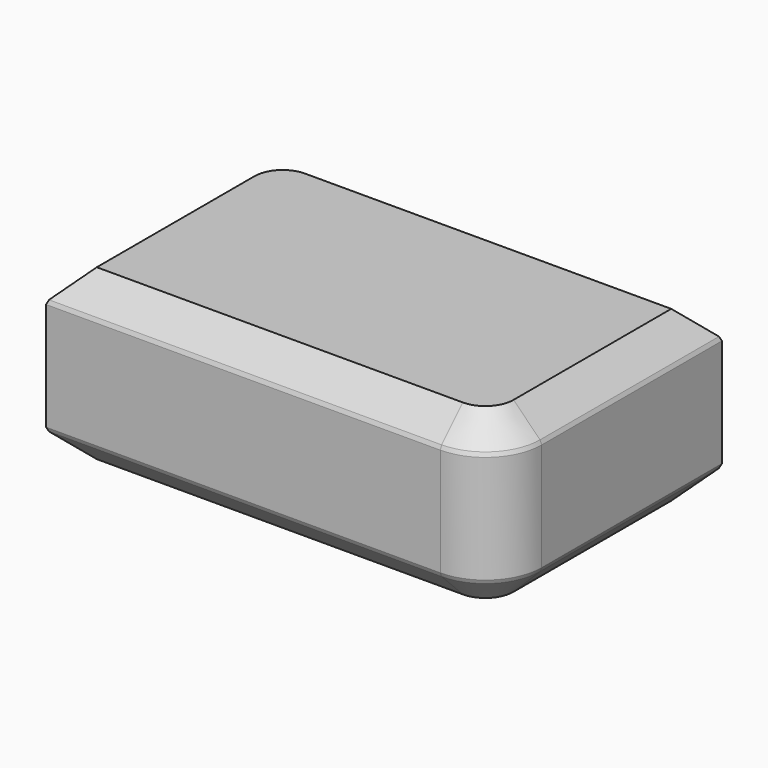
from build123d import *

# Parameters (mm, degrees)
F1_DEPTH     = 76.2
F2_SIZE      = 12.7
F3_T1_DEPTH  = 180.6665699849
F3_T3_DEPTH  = 104.4665699849
F3_T5_DEPTH  = 104.4665699849
F3_T7_DEPTH  = 180.6665699849
F3_T10_ANGLE = 90
F3_T12_ANGLE = 90
F3_T14_ANGLE = 90
F3_T16_ANGLE = 90


# Not quite as in the source:
# - a fillet or chamfer that OpenCascade refuses, or shapes differently, is made with other operations: its cross-section is extruded or revolved along the edge and cut away or added


with BuildPart() as f1:
    # F0 (on Top) → F1 (new body)
    with BuildSketch(Plane.XY):
        with BuildLine():
            Line((137.0133969558, 56.4750247419), (-40.7866030442, 56.4750247419))
            ThreePointArc((-40.7866030442, 56.4750247419), (-58.7471152864, 49.035536984), (-66.1866030442, 31.0750247419))
            Line((-66.1866030442, 31.0750247419), (-66.1866030442, -70.5249752581))
            Line((-66.1866030442, -70.5249752581), (111.6133969558, -70.5249752581))
            ThreePointArc((111.6133969558, -70.5249752581), (129.5739091979, -63.0854875003), (137.0133969558, -45.1249752581))
            Line((137.0133969558, -45.1249752581), (137.0133969558, 56.4750247419))
        make_face()
    extrude(amount=F1_DEPTH)

    # F2
    f2_edges = [f1.edges().sort_by_distance(p)[0] for p in [
        (48.113397, 56.475025, 76.2),
        (-58.747115, 49.035537, 76.2),
        (-66.186603, -19.724975, 76.2),
        (22.713397, -70.524975, 76.2),
        (129.573909, -63.085488, 76.2),
        (137.013397, 5.675025, 76.2),
        (48.113397, 56.475025, 0),
        (-58.747115, 49.035537, 0),
        (-66.186603, -19.724975, 0),
        (22.713397, -70.524975, 0),
        (129.573909, -63.085488, 0),
        (137.013397, 5.675025, 0),
    ]]
    chamfer(f2_edges, length=F2_SIZE)

    # F3: chamfer of 2.54 on 16 edges, made by hand

    # F3_s2 → F3_t1 (cut)
    with BuildSketch(Plane.YZ.offset(-40.7866030442)):
        with BuildLine():
            Line((56.5139053786, 13.8459686089), (55.6921953294, 11.8621850637))
            Line((55.6921953294, 11.8621850637), (55.7281163539, 11.8262640392))
            ThreePointArc((55.7281163539, 11.8262640392), (56.1057846792, 12.2589178883), (56.5109457664, 12.6640789755))
            Line((56.5109457664, 12.6640789755), (56.5258247419, 12.7))
            ThreePointArc((56.5258247419, 12.7), (56.5258247419, 13.2729843045), (56.5647053786, 13.8459686089))
            Line((56.5647053786, 13.8459686089), (56.5139053786, 13.8459686089))
        make_face()
        with BuildLine():
            Line((56.5139053786, 62.3540313911), (55.6921953294, 64.3378149363))
            Line((55.6921953294, 64.3378149363), (55.7281163539, 64.3737359608))
            ThreePointArc((55.7281163539, 64.3737359608), (56.1057846792, 63.9410821117), (56.5109457664, 63.5359210245))
            Line((56.5109457664, 63.5359210245), (56.5258247419, 63.5))
            ThreePointArc((56.5258247419, 63.5), (56.5258247419, 62.9270156955), (56.5647053786, 62.3540313911))
            Line((56.5647053786, 62.3540313911), (56.5139053786, 62.3540313911))
        make_face()
    extrude(amount=F3_T1_DEPTH, mode=Mode.SUBTRACT)

    # F3_s4 → F3_t3 (cut)
    with BuildSketch(Plane.XZ.offset(-59.3415947268)):
        with BuildLine():
            Line((137.0522775925, 13.8459686089), (136.2305675432, 11.8621850637))
            Line((136.2305675432, 11.8621850637), (136.2664885677, 11.8262640392))
            ThreePointArc((136.2664885677, 11.8262640392), (136.644156893, 12.2589178883), (137.0493179802, 12.6640789755))
            Line((137.0493179802, 12.6640789755), (137.0641969558, 12.7))
            ThreePointArc((137.0641969558, 12.7), (137.0641969558, 13.2729843045), (137.1030775925, 13.8459686089))
            Line((137.1030775925, 13.8459686089), (137.0522775925, 13.8459686089))
        make_face()
        with BuildLine():
            Line((137.0522775925, 62.3540313911), (136.2305675432, 64.3378149363))
            Line((136.2305675432, 64.3378149363), (136.2664885677, 64.3737359608))
            ThreePointArc((136.2664885677, 64.3737359608), (136.644156893, 63.9410821117), (137.0493179802, 63.5359210245))
            Line((137.0493179802, 63.5359210245), (137.0641969558, 63.5))
            ThreePointArc((137.0641969558, 63.5), (137.0641969558, 62.9270156955), (137.1030775925, 62.3540313911))
            Line((137.1030775925, 62.3540313911), (137.0522775925, 62.3540313911))
        make_face()
    extrude(amount=F3_T3_DEPTH, mode=Mode.SUBTRACT)

    # F3_s6 → F3_t5 (cut)
    with BuildSketch(Plane.XZ.offset(-31.0750247419)):
        with BuildLine():
            Line((-66.225483681, 13.8459686089), (-65.4037736317, 11.8621850637))
            Line((-65.4037736317, 11.8621850637), (-65.4396946562, 11.8262640392))
            ThreePointArc((-65.4396946562, 11.8262640392), (-65.8173629815, 12.2589178883), (-66.2225240687, 12.6640789755))
            Line((-66.2225240687, 12.6640789755), (-66.2374030442, 12.7))
            ThreePointArc((-66.2374030442, 12.7), (-66.2374030442, 13.2729843045), (-66.276283681, 13.8459686089))
            Line((-66.276283681, 13.8459686089), (-66.225483681, 13.8459686089))
        make_face()
        with BuildLine():
            Line((-66.225483681, 62.3540313911), (-65.4037736317, 64.3378149363))
            Line((-65.4037736317, 64.3378149363), (-65.4396946562, 64.3737359608))
            ThreePointArc((-65.4396946562, 64.3737359608), (-65.8173629815, 63.9410821117), (-66.2225240687, 63.5359210245))
            Line((-66.2225240687, 63.5359210245), (-66.2374030442, 63.5))
            ThreePointArc((-66.2374030442, 63.5), (-66.2374030442, 62.9270156955), (-66.276283681, 62.3540313911))
            Line((-66.276283681, 62.3540313911), (-66.225483681, 62.3540313911))
        make_face()
    extrude(amount=F3_T5_DEPTH, mode=Mode.SUBTRACT)

    # F3_s8 → F3_t7 (cut)
    with BuildSketch(Plane.YZ.offset(-69.0531730292)):
        with BuildLine():
            Line((-70.5638558948, 13.8459686089), (-69.7421458456, 11.8621850637))
            Line((-69.7421458456, 11.8621850637), (-69.7780668701, 11.8262640392))
            ThreePointArc((-69.7780668701, 11.8262640392), (-70.1557351954, 12.2589178883), (-70.5608962826, 12.6640789755))
            Line((-70.5608962826, 12.6640789755), (-70.5757752581, 12.7))
            ThreePointArc((-70.5757752581, 12.7), (-70.5757752581, 13.2729843045), (-70.6146558948, 13.8459686089))
            Line((-70.6146558948, 13.8459686089), (-70.5638558948, 13.8459686089))
        make_face()
        with BuildLine():
            Line((-70.5638558948, 62.3540313911), (-69.7421458456, 64.3378149363))
            Line((-69.7421458456, 64.3378149363), (-69.7780668701, 64.3737359608))
            ThreePointArc((-69.7780668701, 64.3737359608), (-70.1557351954, 63.9410821117), (-70.5608962826, 63.5359210245))
            Line((-70.5608962826, 63.5359210245), (-70.5757752581, 63.5))
            ThreePointArc((-70.5757752581, 63.5), (-70.5757752581, 62.9270156955), (-70.6146558948, 62.3540313911))
            Line((-70.6146558948, 62.3540313911), (-70.5638558948, 62.3540313911))
        make_face()
    extrude(amount=F3_T7_DEPTH, mode=Mode.SUBTRACT)

    # F3_s9 → F3_t10 (revolve, cut)
    with BuildSketch(Plane.YZ.offset(111.6133969558)):
        with BuildLine():
            Line((-70.5638558948, 13.8459686089), (-69.7421458456, 11.8621850637))
            Line((-69.7421458456, 11.8621850637), (-69.7780668701, 11.8262640392))
            ThreePointArc((-69.7780668701, 11.8262640392), (-70.1557351954, 12.2589178883), (-70.5608962826, 12.6640789755))
            Line((-70.5608962826, 12.6640789755), (-70.5757752581, 12.7))
            ThreePointArc((-70.5757752581, 12.7), (-70.5757752581, 13.2729843045), (-70.6146558948, 13.8459686089))
            Line((-70.6146558948, 13.8459686089), (-70.5638558948, 13.8459686089))
        make_face()
    revolve(axis=Axis((111.6133969558, -45.1249752581, 12.7), (0, 0, 1)), revolution_arc=F3_T10_ANGLE, mode=Mode.SUBTRACT)

    # F3_s11 → F3_t12 (revolve, cut)
    with BuildSketch(Plane.YZ.offset(111.6133969558)):
        with BuildLine():
            Line((-70.5638558948, 62.3540313911), (-69.7421458456, 64.3378149363))
            Line((-69.7421458456, 64.3378149363), (-69.7780668701, 64.3737359608))
            ThreePointArc((-69.7780668701, 64.3737359608), (-70.1557351954, 63.9410821117), (-70.5608962826, 63.5359210245))
            Line((-70.5608962826, 63.5359210245), (-70.5757752581, 63.5))
            ThreePointArc((-70.5757752581, 63.5), (-70.5757752581, 62.9270156955), (-70.6146558948, 62.3540313911))
            Line((-70.6146558948, 62.3540313911), (-70.5638558948, 62.3540313911))
        make_face()
    revolve(axis=Axis((111.6133969558, -45.1249752581, 63.5), (0, 0, 1)), revolution_arc=F3_T12_ANGLE, mode=Mode.SUBTRACT)

    # F3_s13 → F3_t14 (revolve, cut)
    with BuildSketch(Plane.YZ.offset(-40.7866030442)):
        with BuildLine():
            Line((56.5139053786, 13.8459686089), (55.6921953294, 11.8621850637))
            Line((55.6921953294, 11.8621850637), (55.7281163539, 11.8262640392))
            ThreePointArc((55.7281163539, 11.8262640392), (56.1057846792, 12.2589178883), (56.5109457664, 12.6640789755))
            Line((56.5109457664, 12.6640789755), (56.5258247419, 12.7))
            ThreePointArc((56.5258247419, 12.7), (56.5258247419, 13.2729843045), (56.5647053786, 13.8459686089))
            Line((56.5647053786, 13.8459686089), (56.5139053786, 13.8459686089))
        make_face()
    revolve(axis=Axis((-40.7866030442, 31.0750247419, 12.7), (0, 0, 1)), revolution_arc=F3_T14_ANGLE, mode=Mode.SUBTRACT)

    # F3_s15 → F3_t16 (revolve, cut)
    with BuildSketch(Plane.YZ.offset(-40.7866030442)):
        with BuildLine():
            Line((56.5139053786, 62.3540313911), (55.6921953294, 64.3378149363))
            Line((55.6921953294, 64.3378149363), (55.7281163539, 64.3737359608))
            ThreePointArc((55.7281163539, 64.3737359608), (56.1057846792, 63.9410821117), (56.5109457664, 63.5359210245))
            Line((56.5109457664, 63.5359210245), (56.5258247419, 63.5))
            ThreePointArc((56.5258247419, 63.5), (56.5258247419, 62.9270156955), (56.5647053786, 62.3540313911))
            Line((56.5647053786, 62.3540313911), (56.5139053786, 62.3540313911))
        make_face()
    revolve(axis=Axis((-40.7866030442, 31.0750247419, 63.5), (0, 0, 1)), revolution_arc=F3_T16_ANGLE, mode=Mode.SUBTRACT)


solid = f1.part
